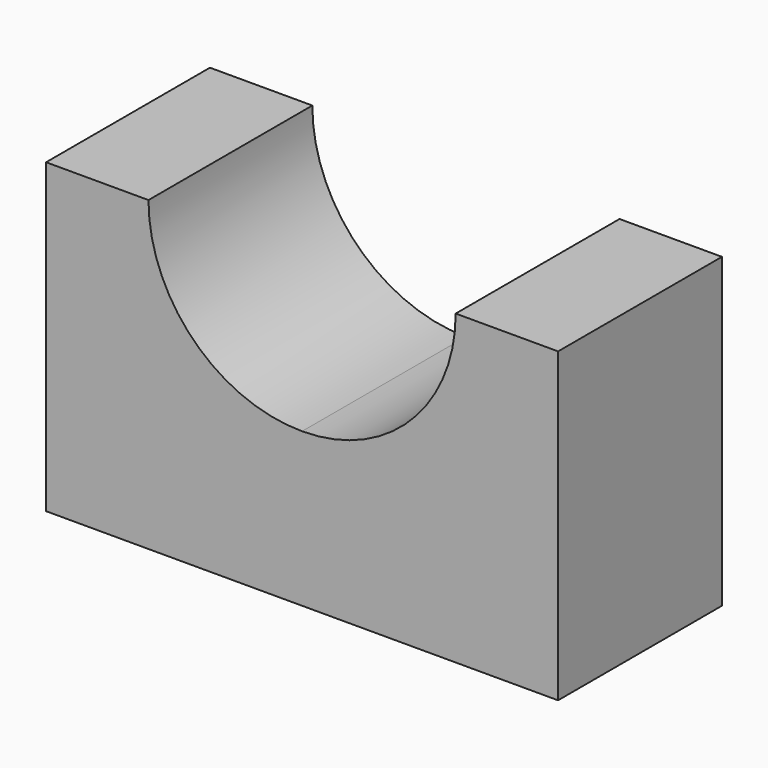
from build123d import *

# Parameters (mm, degrees)
F0_W     = 63.5
F0_H     = 38.1
F1_DEPTH = 25.4
F3_DEPTH = 25.4


with BuildPart() as f1:
    # F0 (on Front) → F1 (new body)
    with BuildSketch(Plane.XZ):
        with Locations((31.75, 19.05)):
            Rectangle(F0_W, F0_H)
    extrude(amount=F1_DEPTH)

    # F2 (on face) → F3 (cut)
    with BuildSketch(Plane.XZ.offset(25.4)):
        with BuildLine():
            Line((49.2131151259, 38.1), (12.7, 38.1))
            ThreePointArc((12.7, 38.1), (18.2796158184, 24.6296158184), (31.75, 19.05))
            ThreePointArc((31.75, 19.05), (45.2203841816, 24.6296158184), (50.8, 38.1))
            Line((50.8, 38.1), (49.2131151259, 38.1))
        make_face()
    extrude(amount=-F3_DEPTH, mode=Mode.SUBTRACT)


solid = f1.part
